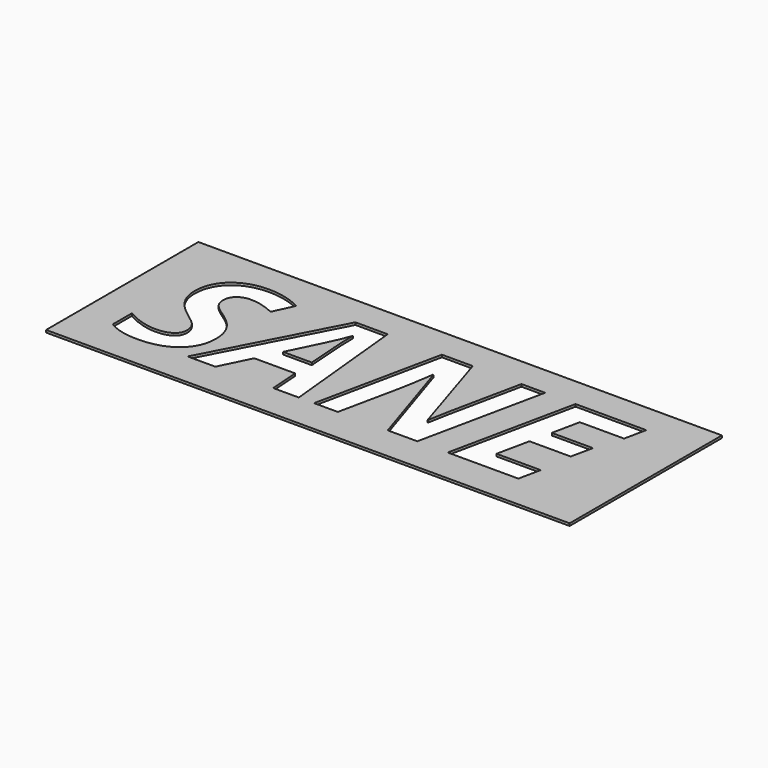
from build123d import *

# Parameters (mm, degrees)
F0_W     = 110
F0_H     = 40
F1_DEPTH = 0.5


# Not quite as in the source:
# - a feature names something its author has since deleted; it is built from what else it names


with BuildPart() as f1:
    # F0 (on Top) → F1 (new body)
    with BuildSketch(Plane.XY):
        Rectangle(F0_W, F0_H)
        with BuildLine():
            add(Edge.make_bspline(
                [(-32.3537972674, -0.9116386363), (-31.2639477814, -2.6641166099), (-31.2639477814, -5.0065664386)],
                knots=[0, 0, 0, 1, 1, 1], degree=2))
            add(Edge.make_bspline(
                [(-31.2639477814, -5.0065664386), (-31.2639477814, -8.8021489153), (-33.9522431803, -11.0109105404)],
                knots=[0, 0, 0, 1, 1, 1], degree=2))
            add(Edge.make_bspline(
                [(-33.9522431803, -11.0109105404), (-36.6405385792, -13.2196721655), (-41.2324377471, -13.2196721655)],
                knots=[0, 0, 0, 1, 1, 1], degree=2))
            add(Edge.make_bspline(
                [(-41.2324377471, -13.2196721655), (-45.2488963864, -13.2196721655), (-47.7017842963, -11.5805385384)],
                knots=[0, 0, 0, 1, 1, 1], degree=2))
            Line((-47.7017842963, -11.5805385384), (-47.7017842963, -6.6050123515))
            add(Edge.make_bspline(
                [(-47.7017842963, -6.6050123515), (-44.1968283492, -8.563835161), (-41.1975625636, -8.563835161)],
                knots=[0, 0, 0, 1, 1, 1], degree=2))
            add(Edge.make_bspline(
                [(-41.1975625636, -8.563835161), (-39.1631768563, -8.563835161), (-38.0181083296, -7.7936748576)],
                knots=[0, 0, 0, 1, 1, 1], degree=2))
            add(Edge.make_bspline(
                [(-38.0181083296, -7.7936748576), (-36.8730398029, -7.0235145541), (-36.8730398029, -5.6808199873)],
                knots=[0, 0, 0, 1, 1, 1], degree=2))
            add(Edge.make_bspline(
                [(-36.8730398029, -5.6808199873), (-36.8730398029, -4.8961283573), (-37.1200723531, -4.3061565022)],
                knots=[0, 0, 0, 1, 1, 1], degree=2))
            add(Edge.make_bspline(
                [(-37.1200723531, -4.3061565022), (-37.3671049033, -3.7161846471), (-37.8204822895, -3.2075882203)],
                knots=[0, 0, 0, 1, 1, 1], degree=2))
            add(Edge.make_bspline(
                [(-37.8204822895, -3.2075882203), (-38.2738596757, -2.6989917934), (-40.0699316287, -1.3562972266)],
                knots=[0, 0, 0, 1, 1, 1], degree=2))
            add(Edge.make_bspline(
                [(-40.0699316287, -1.3562972266), (-42.5809448445, 0.445587257), (-43.5981376982, 2.2067840264)],
                knots=[0, 0, 0, 1, 1, 1], degree=2))
            add(Edge.make_bspline(
                [(-43.5981376982, 2.2067840264), (-44.6153305518, 3.9679807959), (-44.6153305518, 6.0023665032)],
                knots=[0, 0, 0, 1, 1, 1], degree=2))
            add(Edge.make_bspline(
                [(-44.6153305518, 6.0023665032), (-44.6153305518, 8.3448163319), (-43.4876996169, 10.1873885296)],
                knots=[0, 0, 0, 1, 1, 1], degree=2))
            add(Edge.make_bspline(
                [(-43.4876996169, 10.1873885296), (-42.360068682, 12.0299607274), (-40.27918273, 13.0558723769)],
                knots=[0, 0, 0, 1, 1, 1], degree=2))
            add(Edge.make_bspline(
                [(-40.27918273, 13.0558723769), (-38.198296778, 14.0817840264), (-35.4954700526, 14.0817840264)],
                knots=[0, 0, 0, 1, 1, 1], degree=2))
            add(Edge.make_bspline(
                [(-35.4954700526, 14.0817840264), (-31.554574311, 14.0817840264), (-28.2821195875, 12.2857120734)],
                knots=[0, 0, 0, 1, 1, 1], degree=2))
            Line((-28.2821195875, 12.2857120734), (-30.2641925195, 8.0541898022))
            add(Edge.make_bspline(
                [(-30.2641925195, 8.0541898022), (-33.0948949179, 9.3968843691), (-35.4954700526, 9.3968843691)],
                knots=[0, 0, 0, 1, 1, 1], degree=2))
            add(Edge.make_bspline(
                [(-35.4954700526, 9.3968843691), (-37.0009154759, 9.3968843691), (-37.962889289, 8.5802238208)],
                knots=[0, 0, 0, 1, 1, 1], degree=2))
            add(Edge.make_bspline(
                [(-37.962889289, 8.5802238208), (-38.924863102, 7.7635632726), (-38.924863102, 6.4208687058)],
                knots=[0, 0, 0, 1, 1, 1], degree=2))
            add(Edge.make_bspline(
                [(-38.924863102, 6.4208687058), (-38.924863102, 5.3106753627), (-38.326172451, 4.4852960186)],
                knots=[0, 0, 0, 1, 1, 1], degree=2))
            add(Edge.make_bspline(
                [(-38.326172451, 4.4852960186), (-37.7274818, 3.6599166745), (-35.6407833174, 2.2939719853)],
                knots=[0, 0, 0, 1, 1, 1], degree=2))
            add(Edge.make_bspline(
                [(-35.6407833174, 2.2939719853), (-33.4436467535, 0.8408393372), (-32.3537972674, -0.9116386363)],
                knots=[0, 0, 0, 1, 1, 1], degree=2))
        make_face(mode=Mode.SUBTRACT)
        Polygon((-13.0067891911, -12.8534827381), (-13.4427289855, -6.5294494538), (-22.0336492009, -6.5294494538), (-25.1549781289, -12.8534827381), (-30.9675087212, -12.8534827381), (-17.0581230139, 13.8144076192), (-10.2807123433, 13.8144076192), (-7.6127608014, -12.8534827381), align=None, mode=Mode.SUBTRACT)
        with BuildLine():
            Line((22.8913997468, 13.7039695379), (17.2764951946, -12.8534827381))
            Line((17.2764951946, -12.8534827381), (11.0628999915, -12.8534827381))
            Line((11.0628999915, -12.8534827381), (4.5993659729, 7.2346229887))
            Line((4.5993659729, 7.2346229887), (4.4889278916, 7.2346229887))
            Line((4.4889278916, 7.2346229887), (4.4133649939, 6.6533699295))
            add(Edge.make_bspline(
                [(4.4133649939, 6.6533699295), (3.8321119347, 2.7299117797), (3.2159836919, -0.3565419648)],
                knots=[0, 0, 0, 1, 1, 1], degree=2))
            Line((3.2159836919, -0.3565419648), (0.5829073336, -12.8534827381))
            Line((0.5829073336, -12.8534827381), (-4.4100564451, -12.8534827381))
            Line((-4.4100564451, -12.8534827381), (1.1990355764, 13.7039695379))
            Line((1.1990355764, 13.7039695379), (7.6858197174, 13.7039695379))
            Line((7.6858197174, 13.7039695379), (13.8587272064, -5.8610084356))
            Line((13.8587272064, -5.8610084356), (13.9342901041, -5.8610084356))
            add(Edge.make_bspline(
                [(13.9342901041, -5.8610084356), (14.149353736, -4.4776261547), (14.640512571, -1.9172064288)],
                knots=[0, 0, 0, 1, 1, 1], degree=2))
            add(Edge.make_bspline(
                [(14.640512571, -1.9172064288), (15.1316714061, 0.6432132971), (17.9100610292, 13.7039695379)],
                knots=[0, 0, 0, 1, 1, 1], degree=2))
            Line((17.9100610292, 13.7039695379), (22.8913997468, 13.7039695379))
        make_face(mode=Mode.SUBTRACT)
        Polygon((39.4919871183, -8.2034582643), (38.5096694482, -12.8534827381), (23.6702788461, -12.8534827381), (29.2793708677, 13.7039695379), (44.1420115921, 13.7039695379), (43.159693922, 9.0888202477), (33.8596449744, 9.0888202477), (32.63901355, 3.2588520636), (41.3054966631, 3.2588520636), (40.3057414012, -1.3562972266), (31.6450708187, -1.3562972266), (30.1919381706, -8.2034582643), align=None, mode=Mode.SUBTRACT)
    extrude(amount=F1_DEPTH)


with BuildPart() as f1b:
    # F0 (on Top) → F1, piece 2 (new body)
    with BuildSketch(Plane.XY):
        with BuildLine():
            Line((-19.7609497393, -1.8096746128), (-13.7159179233, -1.8096746128))
            Line((-13.7159179233, -1.8096746128), (-14.1867329013, 4.5492338551))
            add(Edge.make_bspline(
                [(-14.1867329013, 4.5492338551), (-14.3669213497, 6.9265588673), (-14.3669213497, 9.141133023)],
                knots=[0, 0, 0, 1, 1, 1], degree=2))
            Line((-14.3669213497, 9.141133023), (-14.3669213497, 9.7979489799))
            add(Edge.make_bspline(
                [(-14.3669213497, 9.7979489799), (-15.1690505714, 7.6182500078), (-16.3489942816, 5.1827996897)],
                knots=[0, 0, 0, 1, 1, 1], degree=2))
            Line((-16.3489942816, 5.1827996897), (-19.7609497393, -1.8096746128))
        make_face()
    extrude(amount=F1_DEPTH)


solid = Compound([f1.part, f1b.part])
